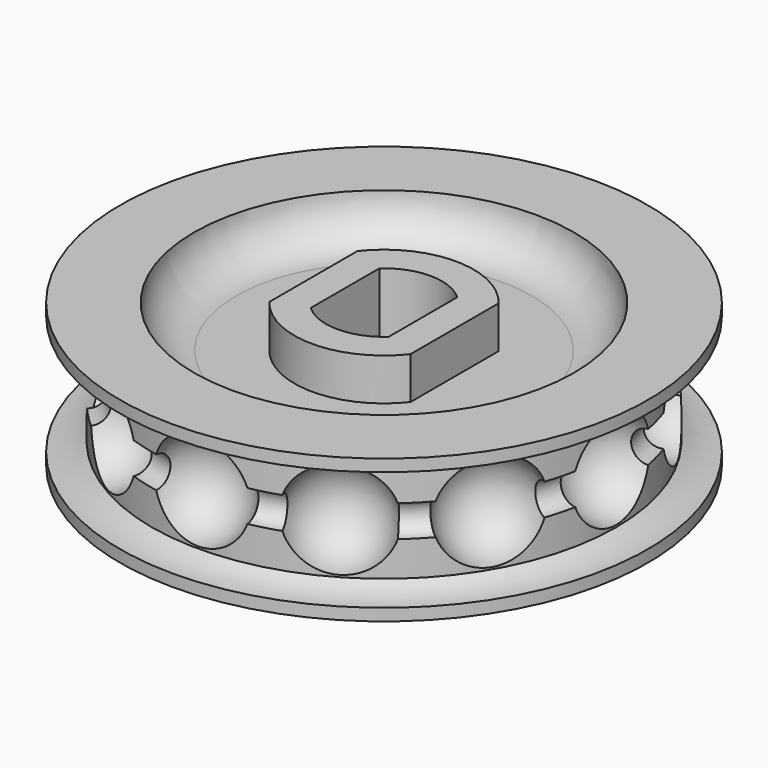
from build123d import *

# Parameters (mm, degrees)
F3_COUNT      = 12
F0_R          = 11.0167051608
F4_DEPTH      = 2.4
F4_DEPTH_BACK = 2.4
F6_R          = 0.75
F12_DEPTH     = 6.801
F13_R         = 9.0167051608
F14_DEPTH     = 2
F17_R         = 1.99999
F18_R         = 1.99999


# Not quite as in the source:
# - a fillet or chamfer is up to 0.001 mm smaller than in the source, because OpenCascade refuses the exact size


with BuildPart() as f2:
    # F1 (on Top) → F2 (revolve)
    with BuildSketch(Plane.XY):
        with BuildLine():
            Line((0, 8.7167051608), (0, 13.3167051608))
            ThreePointArc((0, 13.3167051608), (-2.3, 11.0167051608), (0, 8.7167051608))
        make_face()
    revolve(axis=Axis((0, 11.0167051608, 0), (0, -1, 0)))


with BuildPart() as f3_1:
    # F3: instance of F2
    add(f2.part.rotate(Axis((0, 0, 0), (0, 0, 1)), 1 * 360 / F3_COUNT))


with BuildPart() as f3_2:
    # F3: instance of F2
    add(f2.part.rotate(Axis((0, 0, 0), (0, 0, 1)), 2 * 360 / F3_COUNT))


with BuildPart() as f3_3:
    # F3: instance of F2
    add(f2.part.rotate(Axis((0, 0, 0), (0, 0, 1)), 3 * 360 / F3_COUNT))


with BuildPart() as f3_4:
    # F3: instance of F2
    add(f2.part.rotate(Axis((0, 0, 0), (0, 0, 1)), 4 * 360 / F3_COUNT))


with BuildPart() as f3_5:
    # F3: instance of F2
    add(f2.part.rotate(Axis((0, 0, 0), (0, 0, 1)), 5 * 360 / F3_COUNT))


with BuildPart() as f3_6:
    # F3: instance of F2
    add(f2.part.rotate(Axis((0, 0, 0), (0, 0, 1)), 6 * 360 / F3_COUNT))


with BuildPart() as f3_7:
    # F3: instance of F2
    add(f2.part.rotate(Axis((0, 0, 0), (0, 0, 1)), 7 * 360 / F3_COUNT))


with BuildPart() as f3_8:
    # F3: instance of F2
    add(f2.part.rotate(Axis((0, 0, 0), (0, 0, 1)), 8 * 360 / F3_COUNT))


with BuildPart() as f3_9:
    # F3: instance of F2
    add(f2.part.rotate(Axis((0, 0, 0), (0, 0, 1)), 9 * 360 / F3_COUNT))


with BuildPart() as f3_10:
    # F3: instance of F2
    add(f2.part.rotate(Axis((0, 0, 0), (0, 0, 1)), 10 * 360 / F3_COUNT))


with BuildPart() as f3_11:
    # F3: instance of F2
    add(f2.part.rotate(Axis((0, 0, 0), (0, 0, 1)), 11 * 360 / F3_COUNT))


with BuildPart() as f4:
    # F0 (on Top) → F4 (new body, two sides)
    with BuildSketch(Plane.XY) as f4_sk:
        Circle(F0_R)
    extrude(amount=F4_DEPTH)
    extrude(f4_sk.sketch, amount=-F4_DEPTH_BACK)

    # F5: cut F3_11, F3_10, F3_9, F3_8, F2, F3_1, F3_2, F3_3, F3_4, F3_5, F3_6, F3_7
    add(f3_11.part, mode=Mode.SUBTRACT)
    add(f3_10.part, mode=Mode.SUBTRACT)
    add(f3_9.part, mode=Mode.SUBTRACT)
    add(f3_8.part, mode=Mode.SUBTRACT)
    add(f2.part, mode=Mode.SUBTRACT)
    add(f3_1.part, mode=Mode.SUBTRACT)
    add(f3_2.part, mode=Mode.SUBTRACT)
    add(f3_3.part, mode=Mode.SUBTRACT)
    add(f3_4.part, mode=Mode.SUBTRACT)
    add(f3_5.part, mode=Mode.SUBTRACT)
    add(f3_6.part, mode=Mode.SUBTRACT)
    add(f3_7.part, mode=Mode.SUBTRACT)


with BuildPart() as f7:
    # F6 (on Right) → F7 (revolve)
    with BuildSketch(Plane.YZ):
        with Locations((-11.0167051608, 0)):
            Circle(F6_R)
    revolve(axis=Axis((0, 0, 0), (0, 0, 1)))


with BuildPart() as f4_1:
    add(f4.part)

    # F8: cut F7
    add(f7.part, mode=Mode.SUBTRACT)

    # F9 (on Right) → F10 (revolve)
    with BuildSketch(Plane.YZ):
        with BuildLine():
            Line((0, 3.4), (0, 2.4))
            Line((0, 2.4), (11.0167051608, 2.4))
            ThreePointArc((11.0167051608, 2.4), (11.7364700729, 2.7205207604), (12.5167051608, 2.8301943396))
            Line((12.5167051608, 2.8301943396), (12.5167051608, 3.4))
            Line((12.5167051608, 3.4), (0, 3.4))
        make_face()
        with BuildLine():
            Line((12.5167051608, -3.4), (12.5167051608, -2.8301943396))
            ThreePointArc((12.5167051608, -2.8301943396), (11.7364700729, -2.7205207604), (11.0167051608, -2.4))
            Line((11.0167051608, -2.4), (0, -2.4))
            Line((0, -2.4), (0, -3.4))
            Line((0, -3.4), (12.5167051608, -3.4))
        make_face()
    revolve(axis=Axis((0, 0, 2.9), (0, 0, 1)))

    # F11 (on face) → F12 (cut, through all)
    with BuildSketch(Plane.XY.offset(3.4)):
        with BuildLine():
            Line((1.85, -2.0346989949), (1.85, 2.0346989949))
            ThreePointArc((1.85, 2.0346989949), (0, 2.75), (-1.85, 2.0346989949))
            Line((-1.85, 2.0346989949), (-1.85, -2.0346989949))
            ThreePointArc((-1.85, -2.0346989949), (0, -2.75), (1.85, -2.0346989949))
        make_face()
    extrude(amount=-F12_DEPTH, mode=Mode.SUBTRACT)


with BuildPart() as f14:
    # F13 (on face) → F14 (new body)
    with BuildSketch(Plane(origin=(0, 0, -3.4), x_dir=(1, 0, 0), z_dir=(0, 0, -1))):
        Circle(F13_R)
        with BuildLine():
            ThreePointArc((-3.35, 2.6153393661), (0, 4.25), (3.35, 2.6153393661))
            Line((3.35, 2.6153393661), (3.35, -2.6153393661))
            ThreePointArc((3.35, -2.6153393661), (0, -4.25), (-3.35, -2.6153393661))
            Line((-3.35, -2.6153393661), (-3.35, 2.6153393661))
        make_face(mode=Mode.SUBTRACT)
    extrude(amount=-F14_DEPTH)


with BuildPart() as f15_1:
    # F15: instance of F14
    add(f14.part.mirror(Plane.XY))


with BuildPart() as f4_2:
    add(f4_1.part)

    # F16: cut F14, F15_1
    add(f14.part, mode=Mode.SUBTRACT)
    add(f15_1.part, mode=Mode.SUBTRACT)

    # F17 (radius 2 in the source; OpenCascade refuses exactly that, so slightly less here)
    f17_edges = [f4_2.edges().sort_by_distance(p)[0] for p in [
        (-9.016705, 0, -1.4),
    ]]
    fillet(f17_edges, radius=F17_R)

    # F18 (radius 2 in the source; OpenCascade refuses exactly that, so slightly less here)
    f18_edges = [f4_2.edges().sort_by_distance(p)[0] for p in [
        (-9.016705, 0, 1.4),
    ]]
    fillet(f18_edges, radius=F18_R)


solid = f4_2.part
